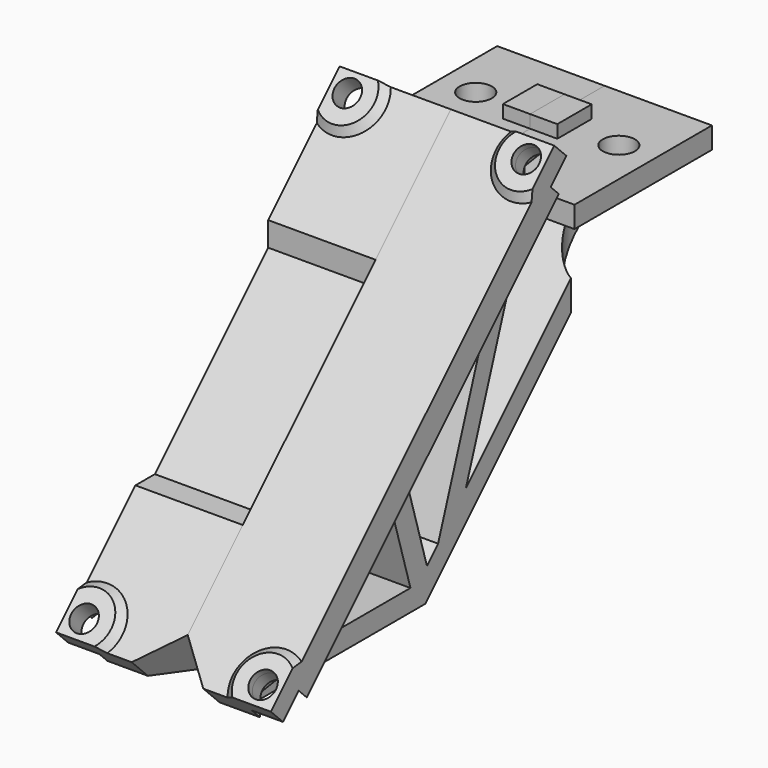
from build123d import *

# Parameters (mm, degrees)
F1_DEPTH      = 15
F2_DEPTH      = 8
F4_DEPTH      = 1.8
F3_R          = 2.25
F5_DEPTH      = 44.3269018078
F6_START      = -3
F6_DEPTH      = 41.3269018078
F7_R          = 1.8
F8_DEPTH      = 4
F9_DEPTH      = 1
F10_T1_DEPTH  = 3
F10_T6_ANGLE  = 249.9440889996
F10_T12_ANGLE = 249.9440889996
F10_T18_DEPTH = 8.7779135172
F10_T24_DEPTH = 9.2748056755
F10_S25_R     = 6.2
F10_T26_DEPTH = 6
F11_R         = 1.8
F12_DEPTH     = 2
F13_T1_DEPTH  = 29.7168298797
F16_DEPTH     = 15


# Not quite as in the source:
# - a fillet or chamfer that OpenCascade refuses, or shapes differently, is made with other operations: its cross-section is extruded or revolved along the edge and cut away or added


with BuildPart() as f1:
    # F0 (on Right) → F1 (new body)
    with BuildSketch(Plane.YZ):
        Polygon((-7, 2.1715728753), (-4, 5.1715728753), (-6.8284271247, 8), (-56.3259018078, -41.4974746831), (-53.4974746831, -44.3259018078), (-50.4974746831, -41.3259018078), (-30.033743948, -20.8621710728), (-27.463730735, -18.2921578598), align=None)
    extrude(amount=F1_DEPTH)



with BuildPart() as f1b:
    # F0 (on Right) → F1, piece 2 (new body)
    with BuildSketch(Plane.YZ):
        Polygon((20, 0), (0, 0), (-4, 0), (-4, -3), (-3.8248562286, -3), (15.7573593129, -3), (20, -3), align=None)
    extrude(amount=F1_DEPTH)


with BuildPart() as f1_1:
    add(f1.part)

    add(f1b.part)  # F2 merges F1b
    # F0 (on Right) → F2 (join)
    with BuildSketch(Plane.YZ):
        Polygon((-21.3259018078, -44.3259018078), (20, -3), (15.7573593129, -3), (-14.2149635258, -32.9723228387), (-3.8248562286, -3), (-4, -3), (-7, -3), (-19.0748035156, -37.8321628285), align=None)
        Polygon((-53.4974746831, -44.3259018078), (-21.3259018078, -44.3259018078), (-19.0748035156, -37.8321628285), (-21.0197849861, -39.777144299), (-27.463730735, -18.2921578598), (-30.033743948, -20.8621710728), (-23.8961012248, -41.3259018078), (-50.4974746831, -41.3259018078), align=None)
        Polygon((-4, -3), (-4, 0), (-4, 5.1715728753), (-7, 2.1715728753), (-7, -3), align=None)
    extrude(amount=F2_DEPTH)

    # F3 (on face) → F4 (join)
    with BuildSketch(Plane.XY):
        Polygon((3.8, 7), (3.8, 10), (3.8, 13), (0, 13), (0, 7), align=None)
    extrude(amount=F4_DEPTH)

    # F3 (on face) → F5 (cut, through all)
    with BuildSketch(Plane.XY):
        with Locations((10, 10)):
            Circle(F3_R)
    extrude(amount=-F5_DEPTH, mode=Mode.SUBTRACT)

    # F3 (on face) → F6 (cut)
    with BuildSketch(Plane.XY.offset(F6_START)):
        with BuildLine():
            Line((15, 6.333939444), (15, 13.666060556))
            ThreePointArc((15, 13.666060556), (8.0712698478, 15.8923679451), (3.8, 10))
            ThreePointArc((3.8, 10), (8.0712698478, 4.1076320549), (15, 6.333939444))
        make_face()
        with Locations((10, 10)):
            Circle(F3_R, mode=Mode.SUBTRACT)
    extrude(amount=-F6_DEPTH, mode=Mode.SUBTRACT)

    # F7 (on face) → F8 (cut, through all)
    with BuildSketch(Plane(origin=(0, -7.4142135624, 7.4142135624), x_dir=(1, 0, 0), z_dir=(0, -0.7071067812, 0.7071067812))):
        with Locations((12.5, -1.6715728753)):
            Circle(F7_R)
        with Locations((12.5, -66.6715728753)):
            Circle(F7_R)
    extrude(amount=-F8_DEPTH, mode=Mode.SUBTRACT)

    # F7 (on face) → F9 (join)
    with BuildSketch(Plane(origin=(0, -7.4142135624, 7.4142135624), x_dir=(1, 0, 0), z_dir=(0, -0.7071067812, 0.7071067812))):
        with BuildLine():
            Line((15, 0.8284271247), (9.6381823957, 0.8284271247))
            ThreePointArc((9.6381823957, 0.8284271247), (9.8129942315, -4.3585786438), (15, -4.5333904795))
            Line((15, -4.5333904795), (15, 0.8284271247))
        make_face()
        with Locations((12.5, -1.6715728753)):
            Circle(F7_R, mode=Mode.SUBTRACT)
        with BuildLine():
            Line((15, -69.1715728753), (15, -63.809755271))
            ThreePointArc((15, -63.809755271), (9.8129942315, -63.9845671067), (9.6381823957, -69.1715728753))
            Line((9.6381823957, -69.1715728753), (15, -69.1715728753))
        make_face()
        with Locations((12.5, -66.6715728753)):
            Circle(F7_R, mode=Mode.SUBTRACT)
    extrude(amount=F9_DEPTH)

    # F10: chamfer of 1 on 5 edges, made by hand

    # F10_s2 → F10_t1 (join)
    with BuildSketch(Plane.XY.offset(-3)):
        Polygon((8, -5), (9, -4), (8, -4), align=None)
    extrude(amount=F10_T1_DEPTH)


with BuildPart() as f10_tool4:
    # F10_s5 → F10_t6 (revolve)
    with BuildSketch(Plane(origin=(11.8343680608, 1.4797429858, 1.4797429858), x_dir=(-0.1240716356, 0.9922732634, 0), z_dir=(0.9847229102, 0.1231275563, 0.1231275563))):
        Polygon((-8.0747037896, 8.1677022303), (-6.6605321208, 8.1568168681), (-7.3730606363, 7.4551737148), align=None)
    revolve(axis=Axis((12.5, -8.5961940777, 6.232233047), (0, -0.7071067812, 0.7071067812)), revolution_arc=F10_T6_ANGLE)

    split(bisect_by=Plane(origin=(0, 0.5857864376, 0.5857864376), x_dir=(1, 0, 0), z_dir=(0, -0.7071067812, -0.7071067812)), keep=Keep.TOP)

    split(bisect_by=Plane.YZ.offset(15), keep=Keep.BOTTOM)


with BuildPart() as f1_2:
    add(f1_1.part)

    # F10_t3: union F10_tool4
    add(f10_tool4.part)


with BuildPart() as f10_tool10:
    # F10_s11 → F10_t12 (revolve)
    with BuildSketch(Plane(origin=(11.8110831902, -47.2300619137, -47.2300619137), x_dir=(0.9701252548, 0.242604596, 0), z_dir=(0.17412866, -0.6963042474, -0.6963042474))):
        Polygon((2.462632391, 12.0869174199), (3.6193556211, 11.2732888997), (2.6341797459, 11.1017415448), align=None)
    revolve(axis=Axis((12.5, -54.5581348548, -39.7297077301), (0, -0.7071067812, 0.7071067812)), revolution_arc=F10_T12_ANGLE)

    split(bisect_by=Plane(origin=(0, -48.9116882454, -48.9116882454), x_dir=(1, 0, 0), z_dir=(0, 0.7071067812, 0.7071067812)), keep=Keep.TOP)

    split(bisect_by=Plane.YZ.offset(15), keep=Keep.BOTTOM)


with BuildPart() as f1_3:
    add(f1_2.part)

    # F10_t9: union F10_tool10
    add(f10_tool10.part)


with BuildPart() as f10_tool16:
    # F10_s17 → F10_t18 (new body)
    with BuildSketch(Plane(origin=(0, -21.0594898175, -21.0594898175), x_dir=(1, 0, 0), z_dir=(0, -0.7071067812, -0.7071067812))):
        Polygon((9, 6.4852813742), (8, 5.4852813742), (8, 6.4852813742), align=None)
    extrude(amount=F10_T18_DEPTH)

    split(bisect_by=Plane(origin=(0, -30.2306117792, -9.0670023373), x_dir=(1, 0, 0), z_dir=(0, -0.9578453043, -0.2872844809)), keep=Keep.TOP)

    split(bisect_by=Plane(origin=(0, -33.295716753, -9.9863126763), x_dir=(1, 0, 0), z_dir=(0, 0.9578453043, 0.2872844809)), keep=Keep.TOP)


with BuildPart() as f1_4:
    add(f1_3.part)

    # F10_t15: union F10_tool16
    add(f10_tool16.part)


with BuildPart() as f10_tool22:
    # F10_s23 → F10_t24 (new body)
    with BuildSketch(Plane.XZ.offset(-22.571682988)):
        Polygon((9, -3), (8, -4), (8, -3), align=None)
    extrude(amount=F10_T24_DEPTH)

    # F10_s25 → F10_t26 (cut, symmetric)
    with BuildSketch(Plane.XY.offset(-3.5)):
        with Locations((10, 10)):
            Circle(F10_S25_R)
    extrude(amount=F10_T26_DEPTH, both=True, mode=Mode.SUBTRACT)

    split(bisect_by=Plane(origin=(0, 11.5, -11.5), x_dir=(1, 0, 0), z_dir=(0, -0.7071067812, 0.7071067812)), keep=Keep.TOP)


with BuildPart() as f1_5:
    add(f1_4.part)

    # F10_t21: union F10_tool22
    add(f10_tool22.part)

    # F11 (on face) → F12 (cut)
    with BuildSketch(Plane(origin=(0, -4.5857864376, 4.5857864376), x_dir=(1, 0, 0), z_dir=(0, 0.7071067812, -0.7071067812))):
        Polygon((10.6524791385, -0.8284271247), (14.3475208615, -0.8284271247), (15, 0.301699894), (15, 3.0414458562), (14.1454482672, 4.5215728751), (10.8545517328, 4.5215728751), (9.2091034656, 1.6715728751), align=None)
        with Locations((12.5, 1.6715728753)):
            Circle(F11_R, mode=Mode.SUBTRACT)
        Polygon((14.1454482672, 63.8215728752), (15, 65.3016998941), (15, 68.0414458563), (14.3475208614, 69.1715728753), (10.6524791386, 69.1715728753), (9.2091034656, 66.6715728752), (10.8545517328, 63.8215728752), align=None)
        with Locations((12.5, 66.6715728753)):
            Circle(F11_R, mode=Mode.SUBTRACT)
        Polygon((14.3475208614, 69.1715728753), (15, 68.0414458563), (15, 69.1715728753), align=None)
        Polygon((15, 0.301699894), (14.3475208615, -0.8284271247), (15, -0.8284271247), align=None)
    extrude(amount=-F12_DEPTH, mode=Mode.SUBTRACT)

    # F13: chamfer of 5 on 1 edges, made by hand

    # F13_s2 → F13_t1 (cut)
    with BuildSketch(Plane(origin=(0, -16.5064859616, 16.5064859616), x_dir=(1, 0, 0), z_dir=(0, 0.7071067812, -0.7071067812))):
        Polygon((0, 64.1715728753), (5, 69.1715728753), (0, 69.1715728753), align=None)
    extrude(amount=F13_T1_DEPTH, mode=Mode.SUBTRACT)


with BuildPart() as f14_1:
    # F14: instance of F1
    add(f1_5.part.mirror(Plane.YZ))

    # F15 (on face) → F16 (cut, through all)
    with BuildSketch(Plane(origin=(-15, 0, 0), x_dir=(0, -1, 0), z_dir=(-1, 0, 0))):
        Polygon((43.1737156777, -28.345288553), (19.9806132548, -5.1521861301), (19.9806132548, -8.5462986798), (39.779603128, -28.345288553), align=None)
    extrude(amount=-F16_DEPTH, mode=Mode.SUBTRACT)


solid = Compound([f1_5.part, f14_1.part])
